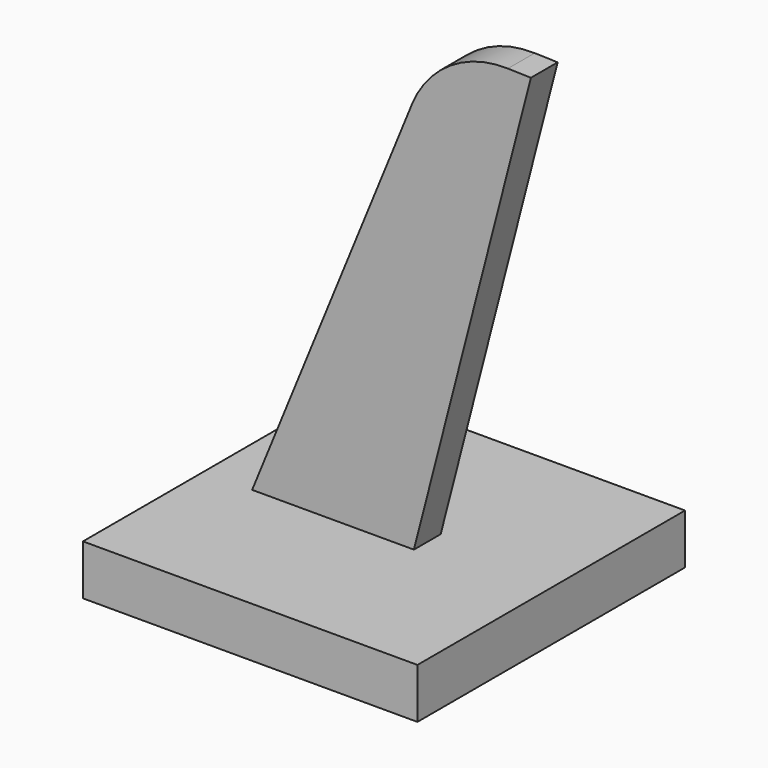
from build123d import *

# Parameters (mm, degrees)
F1_DEPTH = 12.7
F2_DEPTH = 1.27
F3_R     = 7.62


# Not quite as in the source:
# - a feature names something its author has since deleted; it is built from what else it names


with BuildPart() as f1:
    # F0 (on Front) → F1 (new body, symmetric)
    with BuildSketch(Plane.XZ):
        Polygon((-46.139964322, 1.8357970985), (-49.8430333048, 1.8357970985), (-49.8430333048, -1.9742029015), (-24.4430333048, -1.9742029015), (-24.4430333048, 1.8357970985), (-33.8560845901, 1.8357970985), align=None)
    extrude(amount=F1_DEPTH, both=True)

    # F0 (on Front) → F2 (join, symmetric)
    with BuildSketch(Plane.XZ):
        Polygon((-31.998090446, 36.4759527147), (-46.139964322, 1.8357970985), (-33.8560845901, 1.8357970985), (-24.9732534132, 36.2684692324), align=None)
    extrude(amount=F2_DEPTH, both=True)

    # F3
    f3_edges = [f1.edges().sort_by_distance(p)[0] for p in [
        (-31.99809, 0, 36.475953),
    ]]
    fillet(f3_edges, radius=F3_R)


solid = f1.part
